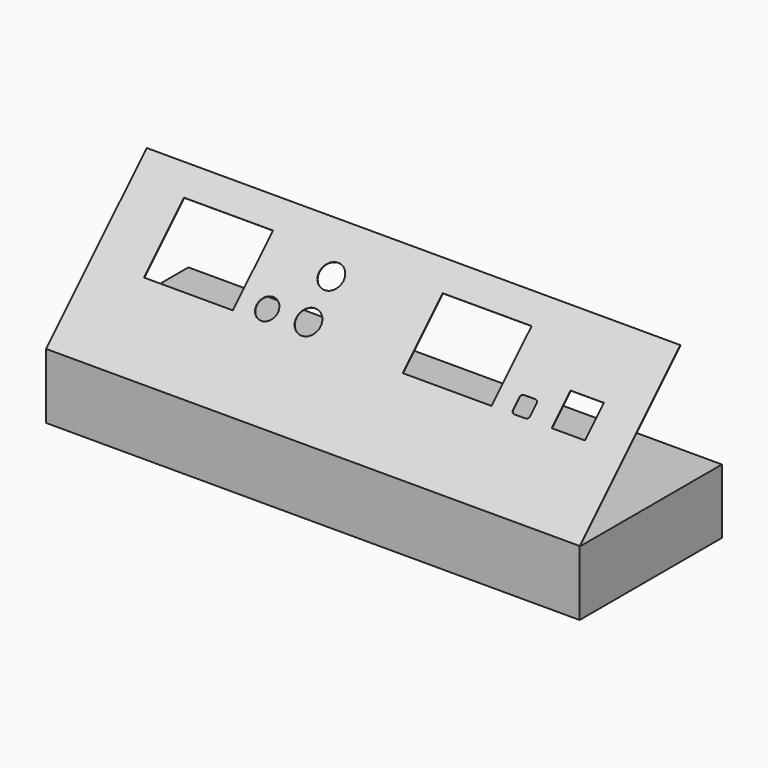
from build123d import *

# Parameters (mm, degrees)
F1_DEPTH = 209.55
F2_W     = 69.85
F2_H     = 55.5625
F2_W_2   = 26.19375
F2_H_2   = 26.19375
F3_DEPTH = 0.4064


# Not quite as in the source:
# - the dataset's text gives a spline's control points without its knots; the knots are read off the source's solid


with BuildPart() as f1:
    # F0 (on Right) → F1 (new body, symmetric)
    with BuildSketch(Plane.YZ):
        Polygon((-139.7, 0), (0, 0), (0, 50.8), (-139.2936, 50.8), (-139.2936, 51.054), (-40.6298144724, 149.7177855276), (-40.9171826682, 150.0051537235), (-139.7, 51.2223363917), align=None)
    extrude(amount=F1_DEPTH, both=True)

    # F2 (on face) → F3 (cut, through all)
    with BuildSketch(Plane(origin=(0, -95.4611681959, 95.4611681959), x_dir=(1, 0, 0), z_dir=(0, -0.7071067812, 0.7071067812))):
        with Locations((-133.4112735748, 28.2945722931)):
            Rectangle(F2_W, F2_H)
        with Locations((69.7887264252, 28.2945722931)):
            Rectangle(F2_W, F2_H)
        with BuildLine():
            add(Edge.make_bspline(
                [(120.8898180252, 13.3087500931), (120.4488486252, 12.8684918931), (120.1918514252, 12.2486810931), (120.1918514252, 11.6258222931)],
                knots=[1, 1, 1, 1, 2, 2, 2, 2], degree=3))
            Line((120.1918514252, 11.6258222931), (120.1918514252, 2.8945722931))
            add(Edge.make_bspline(
                [(120.1918514252, 2.8945722931), (120.1918514252, 2.2706466931), (120.4488486252, 1.6508866931), (120.8898180252, 1.2106284931)],
                knots=[0, 0, 0, 0, 1, 1, 1, 1], degree=3))
            add(Edge.make_bspline(
                [(120.8898180252, 1.2106284931), (121.3304318252, 0.7696590931), (121.9498870252, 0.5133222931), (122.5731014252, 0.5133222931)],
                knots=[1, 1, 1, 1, 2, 2, 2, 2], degree=3))
            Line((122.5731014252, 0.5133222931), (131.3043514252, 0.5133222931))
            add(Edge.make_bspline(
                [(131.3043514252, 0.5133222931), (131.9282516252, 0.5133222931), (132.5476814252, 0.7696590931), (132.9882952252, 1.2106284931)],
                knots=[0, 0, 0, 0, 1, 1, 1, 1], degree=3))
            add(Edge.make_bspline(
                [(132.9882952252, 1.2106284931), (133.4289090252, 1.6508866931), (133.6856014252, 2.2706466931), (133.6856014252, 2.8945722931)],
                knots=[1, 1, 1, 1, 2, 2, 2, 2], degree=3))
            Line((133.6856014252, 2.8945722931), (133.6856014252, 11.6258222931))
            add(Edge.make_bspline(
                [(133.6856014252, 11.6258222931), (133.6856014252, 12.2486810931), (133.4289090252, 12.8684918931), (132.9882952252, 13.3087500931)],
                knots=[0, 0, 0, 0, 1, 1, 1, 1], degree=3))
            add(Edge.make_bspline(
                [(132.9882952252, 13.3087500931), (132.5476814252, 13.7497194931), (131.9282516252, 14.0070722931), (131.3043514252, 14.0070722931)],
                knots=[1, 1, 1, 1, 2, 2, 2, 2], degree=3))
            Line((131.3043514252, 14.0070722931), (122.5731014252, 14.0070722931))
            add(Edge.make_bspline(
                [(122.5731014252, 14.0070722931), (121.9498870252, 14.0070722931), (121.3304318252, 13.7497194931), (120.8898180252, 13.3087500931)],
                knots=[0, 0, 0, 0, 1, 1, 1, 1], degree=3))
        make_face()
        with Locations((165.0387264252, 13.6101972931)):
            Rectangle(F2_W_2, F2_H_2)
        with BuildLine():
            add(Edge.make_bspline(
                [(-70.3677623748, 14.7398368931), (-71.9108123748, 16.2832170931), (-74.0791595748, 17.1820722931), (-76.2612735748, 17.1820722931)],
                knots=[7, 7, 7, 7, 8, 8, 8, 8], degree=3))
            add(Edge.make_bspline(
                [(-76.2612735748, 17.1820722931), (-78.4430573748, 17.1820722931), (-80.6114045748, 16.2832170931), (-82.1544545748, 14.7398368931)],
                knots=[0, 0, 0, 0, 1, 1, 1, 1], degree=3))
            add(Edge.make_bspline(
                [(-82.1544545748, 14.7398368931), (-83.6971997748, 13.1971170931), (-84.5956485748, 11.0291254931), (-84.5956485748, 8.8476972931), (-84.5956485748, 6.6652276931), (-83.6971997748, 4.4972360931), (-82.1544545748, 2.9538304931)],
                knots=[1, 1, 1, 1, 2, 2, 2, 3, 3, 3, 3], degree=3))
            add(Edge.make_bspline(
                [(-82.1544545748, 2.9538304931), (-80.6114045748, 1.4111106931), (-78.4430573748, 0.5133222931), (-76.2612735748, 0.5133222931), (-74.0791595748, 0.5133222931), (-71.9108123748, 1.4111106931), (-70.3677623748, 2.9538304931)],
                knots=[3, 3, 3, 3, 4, 4, 4, 5, 5, 5, 5], degree=3))
            add(Edge.make_bspline(
                [(-70.3677623748, 2.9538304931), (-68.8250171748, 4.4972360931), (-67.9268985748, 6.6652276931), (-67.9268985748, 8.8476972931), (-67.9268985748, 11.0291254931), (-68.8250171748, 13.1971170931), (-70.3677623748, 14.7398368931)],
                knots=[5, 5, 5, 5, 6, 6, 6, 7, 7, 7, 7], degree=3))
        make_face()
        with BuildLine():
            add(Edge.make_bspline(
                [(-37.7754221748, 16.7734878931), (-39.5389695748, 18.5366796931), (-42.0173745748, 19.5633222931), (-44.5112735748, 19.5633222931)],
                knots=[7, 7, 7, 7, 8, 8, 8, 8], degree=3))
            add(Edge.make_bspline(
                [(-44.5112735748, 19.5633222931), (-47.0044867748, 19.5633222931), (-49.4832473748, 18.5366796931), (-51.2464391748, 16.7734878931)],
                knots=[0, 0, 0, 0, 1, 1, 1, 1], degree=3))
            add(Edge.make_bspline(
                [(-51.2464391748, 16.7734878931), (-53.0096563748, 15.0095848931), (-54.0362735748, 12.5315354931), (-54.0362735748, 10.0383222931), (-54.0362735748, 7.5440676931), (-53.0096563748, 5.0653070931), (-51.2464391748, 3.3028010931)],
                knots=[1, 1, 1, 1, 2, 2, 2, 3, 3, 3, 3], degree=3))
            add(Edge.make_bspline(
                [(-51.2464391748, 3.3028010931), (-49.4832473748, 1.5389234931), (-47.0044867748, 0.5133222931), (-44.5112735748, 0.5133222931), (-42.0173745748, 0.5133222931), (-39.5389695748, 1.5389234931), (-37.7754221748, 3.3028010931)],
                knots=[3, 3, 3, 3, 4, 4, 4, 5, 5, 5, 5], degree=3))
            add(Edge.make_bspline(
                [(-37.7754221748, 3.3028010931), (-36.0122303748, 5.0653070931), (-34.9862735748, 7.5440676931), (-34.9862735748, 10.0383222931), (-34.9862735748, 12.5315354931), (-36.0122303748, 15.0095848931), (-37.7754221748, 16.7734878931)],
                knots=[5, 5, 5, 5, 6, 6, 6, 7, 7, 7, 7], degree=3))
        make_face()
        with BuildLine():
            add(Edge.make_bspline(
                [(-37.7754221748, 48.5234878931), (-39.5389695748, 50.2866796931), (-42.0173745748, 51.3133222931), (-44.5112735748, 51.3133222931)],
                knots=[7, 7, 7, 7, 8, 8, 8, 8], degree=3))
            add(Edge.make_bspline(
                [(-44.5112735748, 51.3133222931), (-47.0044867748, 51.3133222931), (-49.4832473748, 50.2866796931), (-51.2464391748, 48.5234878931)],
                knots=[0, 0, 0, 0, 1, 1, 1, 1], degree=3))
            add(Edge.make_bspline(
                [(-51.2464391748, 48.5234878931), (-53.0096563748, 46.7595848931), (-54.0362735748, 44.2815354931), (-54.0362735748, 41.7883222931), (-54.0362735748, 39.2940676931), (-53.0096563748, 36.8153070931), (-51.2464391748, 35.0528010931)],
                knots=[1, 1, 1, 1, 2, 2, 2, 3, 3, 3, 3], degree=3))
            add(Edge.make_bspline(
                [(-51.2464391748, 35.0528010931), (-49.4832473748, 33.2889234931), (-47.0044867748, 32.2633222931), (-44.5112735748, 32.2633222931), (-42.0173745748, 32.2633222931), (-39.5389695748, 33.2889234931), (-37.7754221748, 35.0528010931)],
                knots=[3, 3, 3, 3, 4, 4, 4, 5, 5, 5, 5], degree=3))
            add(Edge.make_bspline(
                [(-37.7754221748, 35.0528010931), (-36.0122303748, 36.8153070931), (-34.9862735748, 39.2940676931), (-34.9862735748, 41.7883222931), (-34.9862735748, 44.2815354931), (-36.0122303748, 46.7595848931), (-37.7754221748, 48.5234878931)],
                knots=[5, 5, 5, 5, 6, 6, 6, 7, 7, 7, 7], degree=3))
        make_face()
    extrude(amount=-F3_DEPTH, mode=Mode.SUBTRACT)


solid = f1.part
